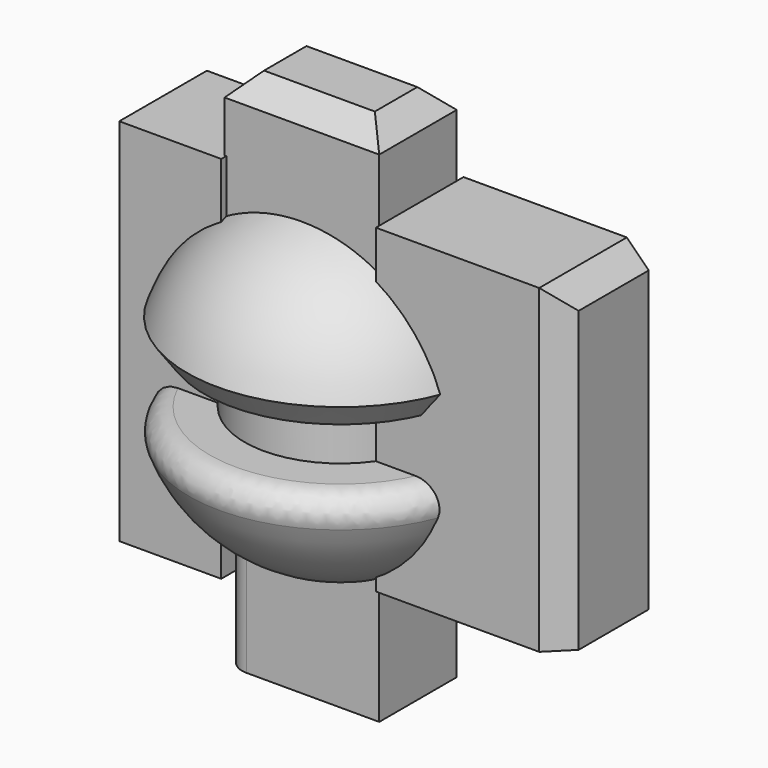
from build123d import *

# Parameters (mm, degrees)
F2_W        = 27.9908
F2_H        = 12.8094828688
F4_W        = 35.8665548265
F4_H        = 22.4658623338
F5_DEPTH    = 60.452
F6_SIZE     = 5.08
F7_T1_DEPTH = 48.5941614915
F8_SIZE     = 5.08
F9_SIZE     = 5.08
F11_R       = 5.08
F12_R       = 5.08
F13_W       = 23.6482750624
F13_H       = 85.7249982655
F14_DEPTH   = 12.7
F15_W       = 42.9610330611
F15_H       = 74.2949992418
F16_DEPTH   = 12.7
F17_SIZE    = 5.08
F18_SIZE    = 5.08


# Not quite as in the source:
# - a fillet or chamfer that OpenCascade refuses, or shapes differently, is made with other operations: its cross-section is extruded or revolved along the edge and cut away or added


with BuildPart() as f1:
    # F0 (on Front) → F1 (revolve)
    with BuildSketch(Plane.XZ):
        with BuildLine():
            Line((0, 37.5782152754), (0, -37.5782152754))
            ThreePointArc((0, -37.5782152754), (37.5782152754, 0), (0, 37.5782152754))
        make_face()
    revolve(axis=Axis((0, 0, 0), (0, 0, -1)))

    # F2 (on Front) → F3 (revolve, cut)
    with BuildSketch(Plane.XZ):
        with Locations((36.2641926143, -0.0985346269)):
            Rectangle(F2_W, F2_H)
    revolve(axis=Axis((0, 0, 0.5912072957), (0, 0, -1)), mode=Mode.SUBTRACT)

    # F4 (on Top) → F5 (join, symmetric)
    with BuildSketch(Plane.XY):
        Rectangle(F4_W, F4_H)
    extrude(amount=F5_DEPTH, both=True)

    # F6
    f6_edges = [f1.edges().sort_by_distance(p)[0] for p in [
        (17.933277, 0, 60.452),
    ]]
    chamfer(f6_edges, length=F6_SIZE)

    # F7: chamfer of 5.08 on 1 edges, made by hand

    # F7_s2 → F7_t1 (cut)
    with BuildSketch(Plane.XZ.offset(-24.2970807458)):
        Polygon((-12.8532774132, 60.452), (-17.9332774132, 55.372), (-17.9332774132, 60.452), align=None)
    extrude(amount=F7_T1_DEPTH, mode=Mode.SUBTRACT)

    # F8
    f8_edges = [f1.edges().sort_by_distance(p)[0] for p in [
        (0, -11.232931, 60.452),
    ]]
    chamfer(f8_edges, length=F8_SIZE)

    # F9
    f9_edges = [f1.edges().sort_by_distance(p)[0] for p in [
        (0, 11.232931, 60.452),
    ]]
    chamfer(f9_edges, length=F9_SIZE)

    # F10: chamfer of 5.08 on 1 edges, made by hand

    # F10_s1 → F10_t2 (revolve, cut)
    with BuildSketch(Plane.XZ):
        with BuildLine():
            Line((35.7430389368, 12.1242465057), (31.4404153436, 6.1412357976))
            Line((31.4404153436, 6.1412357976), (31.4404153436, 6.0396357976))
            ThreePointArc((31.4404153436, 6.0396357976), (34.2428560987, 6.2046068075), (37.0452968537, 6.2046068075))
            Line((37.0452968537, 6.2046068075), (37.1454560053, 6.3232568618))
            ThreePointArc((37.1454560053, 6.3232568618), (36.5270685447, 9.2488779166), (35.8393564224, 12.1565807287))
            Line((35.8393564224, 12.1565807287), (35.7430389368, 12.1242465057))
        make_face()
    revolve(axis=Axis((0, 0, 6.3062068075), (0, 0, 1)), mode=Mode.SUBTRACT)

    # F11
    f11_edges = [f1.edges().sort_by_distance(p)[0] for p in [
        (-37.01121, 0, -6.503276),
    ]]
    fillet(f11_edges, radius=F11_R)

    # F12
    f12_edges = [f1.edges().sort_by_distance(p)[0] for p in [
        (-17.933277, -11.232931, -45.752921),
    ]]
    fillet(f12_edges, radius=F12_R)


with BuildPart() as f14:
    # F13 (on Front) → F14 (new body, symmetric)
    with BuildSketch(Plane.XZ):
        with Locations((-29.3632755056, 0.6897393614)):
            Rectangle(F13_W, F13_H)
    extrude(amount=F14_DEPTH, both=True)


with BuildPart() as f16:
    # F15 (on Front) → F16 (new body, symmetric)
    with BuildSketch(Plane.XZ):
        with Locations((39.8079296574, 4.0399134159)):
            Rectangle(F15_W, F15_H)
    extrude(amount=F16_DEPTH, both=True)

    # F17
    f17_edges = [f16.edges().sort_by_distance(p)[0] for p in [
        (61.288446, 0, 41.187413),
    ]]
    chamfer(f17_edges, length=F17_SIZE)

    # F18
    f18_edges = [f16.edges().sort_by_distance(p)[0] for p in [
        (61.288446, -12.7, 1.499913),
    ]]
    chamfer(f18_edges, length=F18_SIZE)


solid = Compound([f1.part, f14.part, f16.part])
